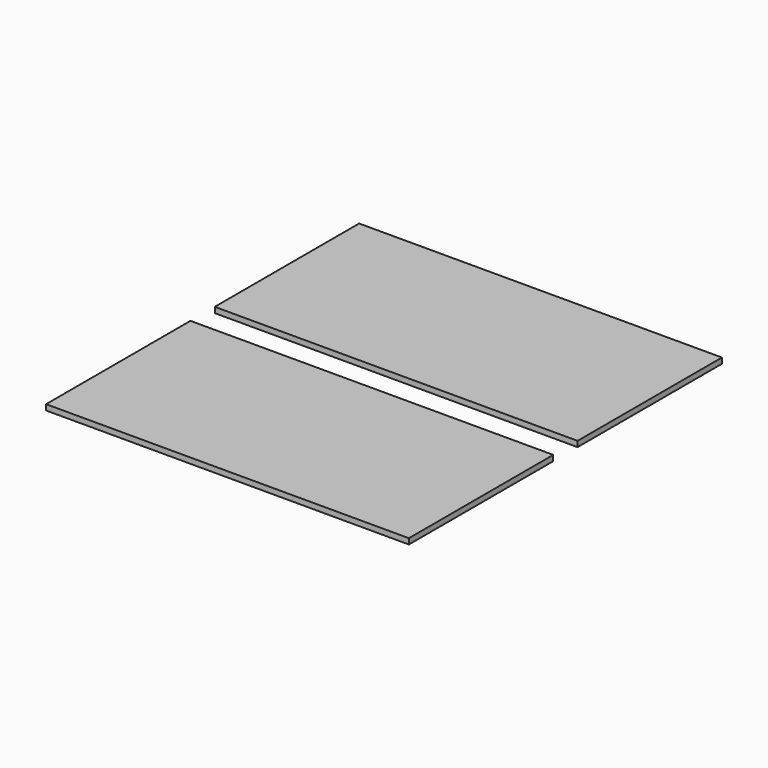
from build123d import *

# Parameters (mm, degrees)
F0_W     = 1212.85
F0_H     = 603.25
F1_DEPTH = 18.6436


# Not quite as in the source:
# - the program builds the solid bodies; features that only make, move or delete a surface that nothing else refers to are left out


with BuildPart() as f1:
    # F0 (on Top) → F1 (new body)
    with BuildSketch(Plane.XY):
        Rectangle(F0_W, F0_H)
    extrude(amount=F1_DEPTH)


with BuildPart() as f1b:
    # F0 (on Top) → F1, piece 2 (new body)
    with BuildSketch(Plane.XY):
        with Locations((0, -704.85)):
            Rectangle(F0_W, F0_H)
    extrude(amount=F1_DEPTH)


solid = Compound([f1.part, f1b.part])
